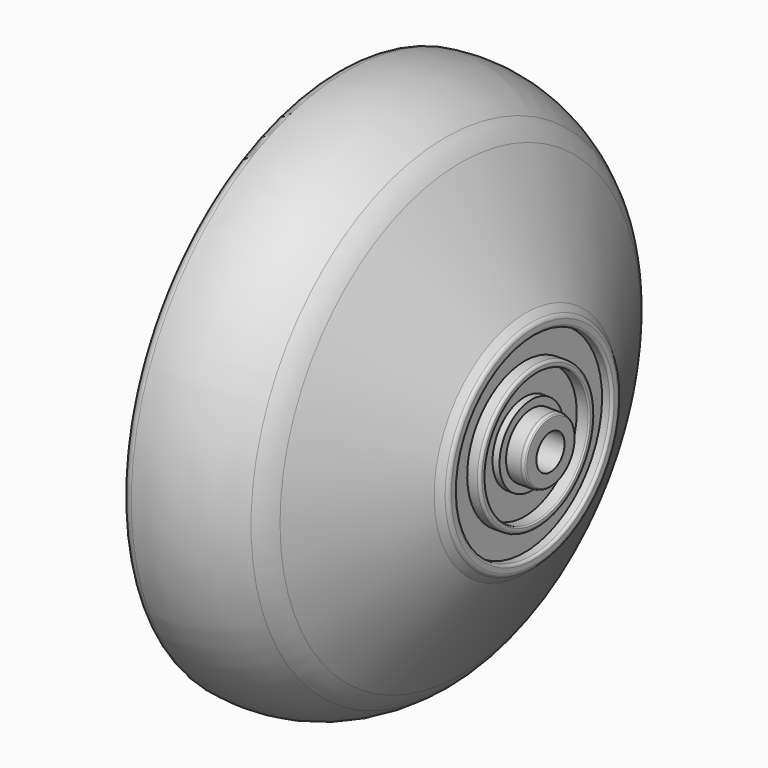
from build123d import *


# Not quite as in the source:
# - ends of sketch curves that miss each other by under 0.0002 mm in the source are joined


with BuildPart() as f1:
    # F0 (on Front) → F1 (revolve)
    with BuildSketch(Plane.XZ):
        with BuildLine():
            ThreePointArc((2.673171, 10.3908833116), (2.5925072418, 10.6420979852), (2.3806730751, 10.7993930578))
            Line((2.3806730751, 10.7993930578), (1.7919312704, 11.417709443))
            Line((1.7919312704, 11.417709443), (-4.7289006394, 22.4696731633))
            ThreePointArc((-4.7289006394, 22.4696731633), (-5.4053057585, 23.4019298626), (-6.245015962, 24.1902909553))
            ThreePointArc((-6.245015962, 24.1902909553), (-10.8844153273, 26.4988051942), (-16.0549171269, 26.8440233886))
            ThreePointArc((-16.0549171269, 26.8440233886), (-17.0816074298, 25.8173330858), (-16.0549171269, 24.790642783))
            ThreePointArc((-16.0549171269, 24.790642783), (-13.5976320817, 22.8564021798), (-12.1680862278, 20.0750472662))
            ThreePointArc((-12.1680862278, 20.0750472662), (-11.7319634551, 19.4206195391), (-10.9873679122, 19.167526275))
            Line((-10.9873679122, 19.167526275), (-5.5484585347, 19.167526275))
            ThreePointArc((-5.5484585347, 19.167526275), (-4.6301064326, 18.9205258244), (-3.9595614905, 18.246174813))
            Line((-3.9595614905, 18.246174813), (-0.8720830878, 12.8515981778))
            ThreePointArc((-0.8720830878, 12.8515981778), (0.0660653596, 10.5178290481), (0.3347051314, 8.0169424987))
            Line((0.3347051314, 8.0169424987), (0.2124717155, 4.0234341655))
            ThreePointArc((0.2124717155, 4.0234341655), (0.0523024795, 3.124834336), (-0.4084772998, 2.3369143954))
            ThreePointArc((-0.4084772998, 2.3369143954), (-1.2026479798, 1.2699423116), (-1.5981009122, 0))
            Line((-1.5981009122, 0), (0, 0))
            Line((0, 0), (1.054421, 1.754851))
            Line((1.054421, 1.754851), (4.24833, 1.754851))
            Line((4.24833, 1.754851), (4.24833, 2.965108))
            ThreePointArc((4.24833, 2.965108), (4.2243561549, 3.0393632641), (4.1614868664, 3.085580599))
            Line((4.1614868664, 3.085580599), (3.879268, 3.179662))
            ThreePointArc((3.879268, 3.179662), (3.8594525644, 3.1845473579), (3.83911, 3.18619))
            Line((3.83911, 3.18619), (2.36708, 3.18619))
            Line((2.36708, 3.18619), (2.36708, 3.998))
            Line((2.36708, 3.998), (1.672421, 3.998))
            Line((1.672421, 3.998), (1.672421, 6.492))
            Line((1.672421, 6.492), (2.801421, 6.492))
            ThreePointArc((2.801421, 6.492), (2.8912235612, 6.5291974388), (2.928421, 6.619))
            Line((2.928421, 6.619), (2.928421, 6.896))
            ThreePointArc((2.928421, 6.896), (2.8540261224, 7.0756051224), (2.674421, 7.15))
            Line((2.674421, 7.15), (1.668421, 7.15))
            Line((1.668421, 7.15), (1.668421, 7.150491))
            Line((1.668421, 7.150491), (1.668421, 9.65))
            Line((1.668421, 9.65), (1.668421, 9.65036))
            Line((1.668421, 9.65036), (2.419171, 9.651342))
            ThreePointArc((2.419171, 9.651342), (2.5987761224, 9.7257368776), (2.673171, 9.905342))
            Line((2.673171, 9.905342), (2.673171, 10.3908833116))
        make_face()
    revolve(axis=Axis((-0.7990504561, 0, 0), (-1, 0, 0)))


solid = f1.part
